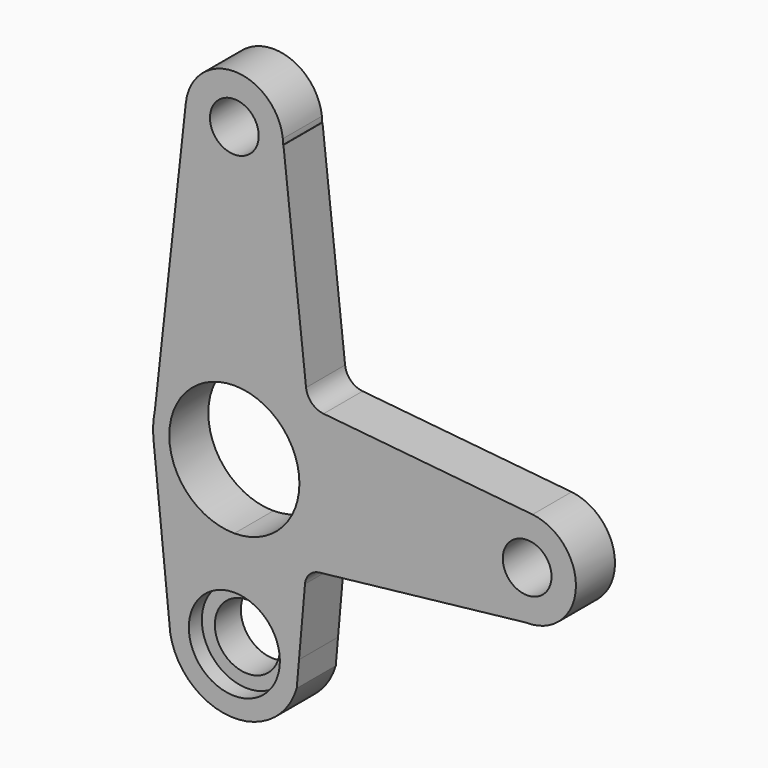
from build123d import *

# Parameters (mm, degrees)
F1_DEPTH = 15
F3_START = 10
F2_R     = 14
F3_DEPTH = 15


with BuildPart() as f1:
    # F0 (on Front) → F1 (new body)
    with BuildSketch(Plane.XZ):
        with BuildLine():
            Line((-24.8721406347, 47.4748029292), (-19.9908943662, -0.603442158))
            Line((-19.9908943662, -0.603442158), (-19.7042578352, -3.4266927442))
            ThreePointArc((-19.7042578352, -3.4266927442), (-1.1601406694, -19.966323488), (19.1747802681, -5.6857542744))
            Line((19.1747802681, -5.6857542744), (19.8706965994, 2.2705542616))
            Line((19.8706965994, 2.2705542616), (21.7154896457, 23.361800439))
            ThreePointArc((21.7154896457, 23.361800439), (23.1184617772, 26.4186682546), (26.1405225938, 27.895123491))
            Line((26.1405225938, 27.895123491), (89.6744252597, 35.0035337133))
            ThreePointArc((89.6744252597, 35.0035337133), (104.9669737345, 49.0051647211), (91.6621115435, 64.9076284236))
            Line((91.6621115435, 64.9076284236), (27.4153419388, 71.2848644166))
            ThreePointArc((27.4153419388, 71.2848644166), (23.7872845646, 72.9910681825), (22.0437681238, 76.6013426904))
            Line((22.0437681238, 76.6013426904), (15.089959345, 140))
            Line((15.089959345, 140), (15, 140))
            ThreePointArc((15, 140), (14.9776275535, 140.8189461935), (14.910576951, 141.6354494764))
            ThreePointArc((14.910576951, 141.6354494764), (0.0042894025, 154.9999993867), (-14.9096391656, 141.6439768707))
            Line((-14.9096391656, 141.6439768707), (-24.4285254093, 55.3148066248))
            ThreePointArc((-24.4285254093, 55.3148066248), (-24.960074773, 51.4123310642), (-24.8721406347, 47.4748029292))
        make_face()
        with BuildLine():
            ThreePointArc((10, 0), (-7.0710678119, -7.0710678119), (0, 10))
            ThreePointArc((0, 10), (7.0710678119, 7.0710678119), (10, 0))
        make_face(mode=Mode.SUBTRACT)
        with BuildLine():
            ThreePointArc((0, 30), (-20, 50), (0, 70))
            ThreePointArc((0, 70), (14.1421356237, 64.1421356237), (20, 50))
            ThreePointArc((20, 50), (14.1421356237, 35.8578643763), (0, 30))
        make_face(mode=Mode.SUBTRACT)
        with BuildLine():
            ThreePointArc((97.5, 50), (90, 42.5), (82.5, 50))
            ThreePointArc((82.5, 50), (90, 57.5), (97.5, 50))
        make_face(mode=Mode.SUBTRACT)
        with BuildLine():
            ThreePointArc((0, 132.5), (-5.3033008589, 145.3033008589), (7.5, 140))
            ThreePointArc((7.5, 140), (5.3033008589, 134.6966991411), (0, 132.5))
        make_face(mode=Mode.SUBTRACT)
    extrude(amount=F1_DEPTH)

    # F2 (on Front) → F3 (cut)
    with BuildSketch(Plane.XZ.offset(F3_START)):
        Circle(F2_R)
    extrude(amount=F3_DEPTH, mode=Mode.SUBTRACT)


solid = f1.part
